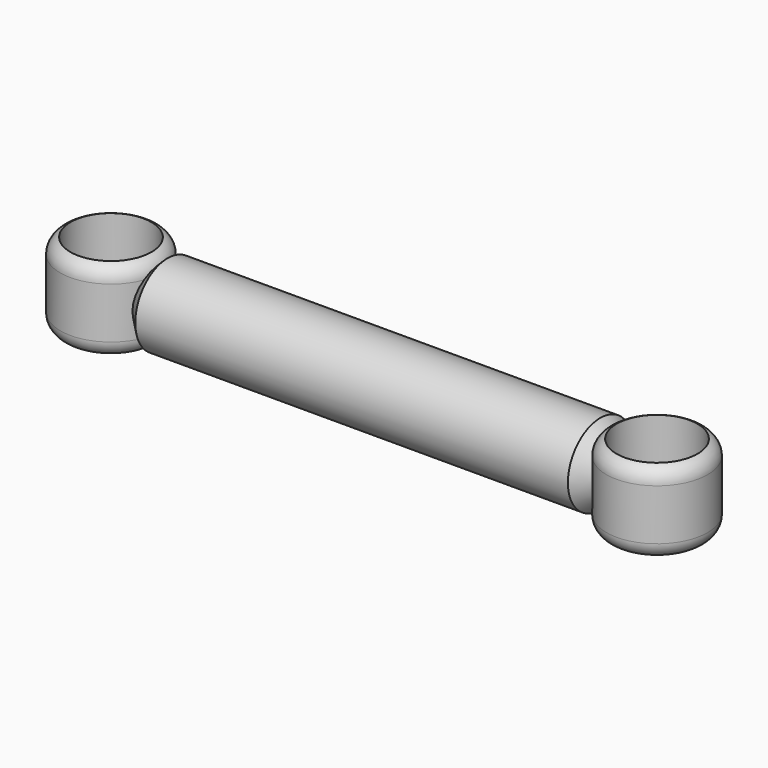
from build123d import *

# Parameters (mm, degrees)
F0_R          = 15.875
F0_R_2        = 12.7
F1_DEPTH      = 12.7
F3_R          = 12.7
F5_2_T2_ANGLE = 180
F5_2_T4_ANGLE = 180
F5_2_T6_ANGLE = 180
F5_2_T8_ANGLE = 180
F6_SIZE       = 5.08


# Not quite as in the source:
# - a fillet or chamfer that OpenCascade refuses, or shapes differently, is made with other operations: its cross-section is extruded or revolved along the edge and cut away or added


with BuildPart() as f1:
    # F0 (on Top) → F1 (new body, symmetric)
    with BuildSketch(Plane.XY):
        Circle(F0_R)
        Circle(F0_R_2, mode=Mode.SUBTRACT)
    extrude(amount=F1_DEPTH, both=True)

    # F5: fillet of radius 5.08 on 2 edges, made by hand

    # F5_s1 → F5_t2 (revolve, cut)
    with BuildSketch(Plane.XZ):
        with BuildLine():
            ThreePointArc((15.875, 7.9907139607), (15.0071134838, 10.8305202921), (12.7, 12.7))
            Line((12.7, 12.7), (15.875, 12.7))
            Line((15.875, 12.7), (15.875, 7.9907139607))
        make_face()
    revolve(axis=Axis((0, 0, 12.7), (0, 0, 1)), mode=Mode.SUBTRACT)

    # F5_s3 → F5_t4 (revolve, cut)
    with BuildSketch(Plane.XZ):
        with BuildLine():
            ThreePointArc((15.875, -7.9907139607), (15.0071134838, -10.8305202921), (12.7, -12.7))
            Line((12.7, -12.7), (15.875, -12.7))
            Line((15.875, -12.7), (15.875, -7.9907139607))
        make_face()
    revolve(axis=Axis((0, 0, -12.7), (0, 0, 1)), mode=Mode.SUBTRACT)


with BuildPart() as f1b:
    # F0 (on Top) → F1, piece 2 (new body, symmetric)
    with BuildSketch(Plane.XY):
        with BuildLine():
            ThreePointArc((186.9948, 0), (171.1198, 15.875), (155.2448, 0))
            ThreePointArc((155.2448, 0), (171.1198, -15.875), (186.9948, 0))
        make_face()
        with BuildLine():
            ThreePointArc((183.8198, 0), (171.1198, -12.7), (158.4198, 0))
            ThreePointArc((158.4198, 0), (171.1198, 12.7), (183.8198, 0))
        make_face(mode=Mode.SUBTRACT)
    extrude(amount=F1_DEPTH, both=True)

    # F5#2: fillet of radius 5.08 on 4 edges, made by hand

    # F5_2_s1 → F5_2_t2 (revolve, cut)
    with BuildSketch(Plane.XZ):
        with BuildLine():
            ThreePointArc((186.9948, 7.9907139607), (186.1269134838, 10.8305202921), (183.8198, 12.7))
            Line((183.8198, 12.7), (186.9948, 12.7))
            Line((186.9948, 12.7), (186.9948, 7.9907139607))
        make_face()
    revolve(axis=Axis((171.1198, 0, 12.7), (0, 0, 1)), revolution_arc=F5_2_T2_ANGLE, mode=Mode.SUBTRACT)

    # F5_2_s3 → F5_2_t4 (revolve, cut)
    with BuildSketch(Plane.XZ):
        with BuildLine():
            ThreePointArc((155.2448, 7.9907139607), (156.1126865162, 10.8305202921), (158.4198, 12.7))
            Line((158.4198, 12.7), (155.2448, 12.7))
            Line((155.2448, 12.7), (155.2448, 7.9907139607))
        make_face()
    revolve(axis=Axis((171.1198, 0, 12.7), (0, 0, 1)), revolution_arc=F5_2_T4_ANGLE, mode=Mode.SUBTRACT)

    # F5_2_s5 → F5_2_t6 (revolve, cut)
    with BuildSketch(Plane.XZ):
        with BuildLine():
            ThreePointArc((186.9948, -7.9907139607), (186.1269134838, -10.8305202921), (183.8198, -12.7))
            Line((183.8198, -12.7), (186.9948, -12.7))
            Line((186.9948, -12.7), (186.9948, -7.9907139607))
        make_face()
    revolve(axis=Axis((171.1198, 0, -12.7), (0, 0, 1)), revolution_arc=F5_2_T6_ANGLE, mode=Mode.SUBTRACT)

    # F5_2_s7 → F5_2_t8 (revolve, cut)
    with BuildSketch(Plane.XZ):
        with BuildLine():
            ThreePointArc((155.2448, -7.9907139607), (156.1126865162, -10.8305202921), (158.4198, -12.7))
            Line((158.4198, -12.7), (155.2448, -12.7))
            Line((155.2448, -12.7), (155.2448, -7.9907139607))
        make_face()
    revolve(axis=Axis((171.1198, 0, -12.7), (0, 0, 1)), revolution_arc=F5_2_T8_ANGLE, mode=Mode.SUBTRACT)


with BuildPart() as f4:
    # F4: sweep along a path in F0
    with BuildLine(Plane.XY) as f4_path:
        Line((12.7, 0), (15.875, 0))
        Line((15.875, 0), (155.2448, 0))
        Line((155.2448, 0), (158.4198, 0))
    # F3 (on offset) → F4 (sweep)
    with BuildSketch(Plane.YZ.offset(12.7)):
        Circle(F3_R)
    sweep(path=f4_path.line)

    # F6
    f6_edges = [f4.edges().sort_by_distance(p)[0] for p in [
        (158.4198, -12.7, 0),
        (12.7, -12.7, 0),
    ]]
    chamfer(f6_edges, length=F6_SIZE)


solid = Compound([f1.part, f1b.part, f4.part])
